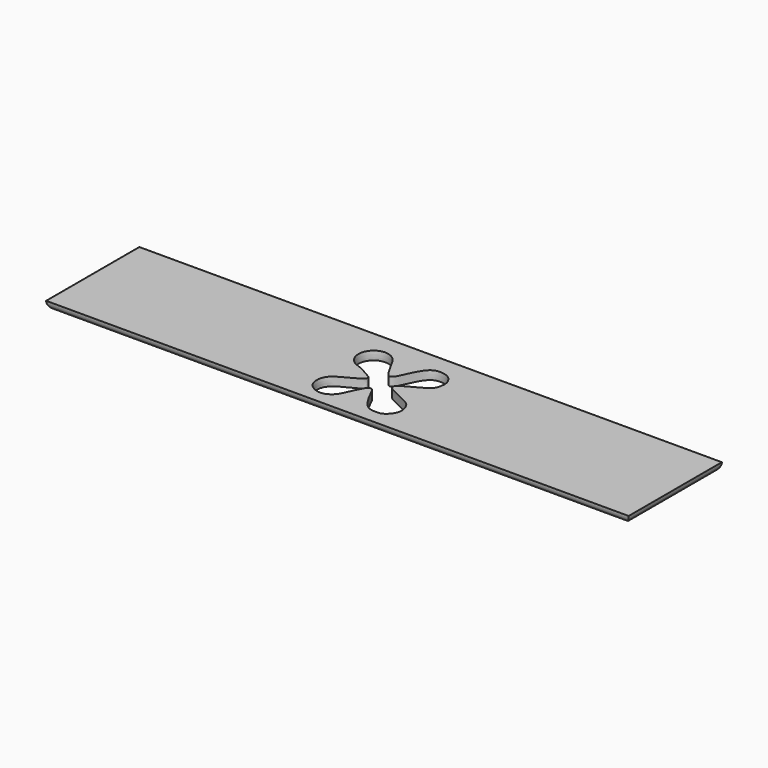
from build123d import *

# Parameters (mm, degrees)
F0_W        = 1282.7
F0_H        = 256.54
F1_DEPTH    = 19.1262
F2_R        = 19.0590813946
F3_T1_DEPTH = 1291.926483958
F3_T3_DEPTH = 265.766483958
F6_DEPTH    = 219.27551


# Not quite as in the source:
# - a fillet or chamfer that OpenCascade refuses, or shapes differently, is made with other operations: its cross-section is extruded or revolved along the edge and cut away or added


with BuildPart() as f1:
    # F0 (on Top) → F1 (new body)
    with BuildSketch(Plane.XY):
        with Locations((1.9049979746, -79.4771378769)):
            Rectangle(F0_W, F0_H)
    extrude(amount=F1_DEPTH)

    # F2
    f2_edges = [f1.edges().sort_by_distance(p)[0] for p in [
        (1.904998, -207.747138, 0),
        (-639.445002, -79.477138, 0),
        (1.904998, 48.792862, 0),
        (643.254998, -79.477138, 0),
    ]]
    fillet(f2_edges, radius=F2_R)

    # F3: fillet of radius 25.4 on 5 edges, made by hand

    # F3_s2 → F3_t1 (cut)
    with BuildSketch(Plane.YZ.offset(-644.0582440044)):
        with BuildLine():
            ThreePointArc((48.7928621231, 19.0590813946), (47.8708238484, 19.1094148025), (46.9475653315, 19.1262))
            Line((46.9475653315, 19.1262), (48.7928621231, 19.1262))
            Line((48.7928621231, 19.1262), (48.7928621231, 19.0590813946))
        make_face()
        with BuildLine():
            ThreePointArc((-205.9018410853, 19.1262), (-206.8250996022, 19.1094148025), (-207.7471378769, 19.0590813946))
            Line((-207.7471378769, 19.0590813946), (-207.7471378769, 19.1262))
            Line((-207.7471378769, 19.1262), (-205.9018410853, 19.1262))
        make_face()
    extrude(amount=F3_T1_DEPTH, mode=Mode.SUBTRACT)

    # F3_s4 → F3_t3 (cut)
    with BuildSketch(Plane.XZ.offset(-53.4061041021)):
        with BuildLine():
            ThreePointArc((-637.5997052338, 19.1262), (-638.5229637507, 19.1094148025), (-639.4450020254, 19.0590813946))
            Line((-639.4450020254, 19.0590813946), (-639.4450020254, 19.1262))
            Line((-639.4450020254, 19.1262), (-637.5997052338, 19.1262))
        make_face()
        with BuildLine():
            ThreePointArc((643.2549979746, 19.0590813946), (642.3329597, 19.1094148025), (641.409701183, 19.1262))
            Line((641.409701183, 19.1262), (643.2549979746, 19.1262))
            Line((643.2549979746, 19.1262), (643.2549979746, 19.0590813946))
        make_face()
    extrude(amount=F3_T3_DEPTH, mode=Mode.SUBTRACT)

    # F5 (on face) → F6 (cut)
    with BuildSketch(Plane.XY.offset(19.1262)):
        with BuildLine():
            add(Edge.make_bspline(
                [(-3.9519034326, -58.3399571478), (-6.0360933822, -57.4592299023), (-12.1793255374, -50.9473924507), (-26.2298304514, -24.3224308517), (-41.2097493794, 2.9789491334), (-72.4360201049, 10.037217761), (-96.3421712705, -9.9579243998), (-97.7950455083, -37.9438595198), (-81.6831294585, -58.938620379), (-61.293313593, -63.2792187165), (-36.9211355632, -78.9844871293), (-29.9788714537, -81.7077400378), (-25.2014666644, -91.8610913919), (-59.0203507366, -108.463960156), (-80.1276897444, -119.4826575733), (-93.5746327257, -137.4339169363), (-90.7677488387, -163.9002438236), (-75.433428627, -176.9677968773), (-53.4410245485, -183.5763107426), (-29.7456035179, -168.6651562344), (-22.0503636386, -143.9154043667), (-9.3604006708, -122.623140043), (-5.8408588762, -114.5198839058), (0.1862852859, -112.8583130861), (6.0845539399, -116.437681633), (11.1546658823, -128.0348941145), (35.0716542184, -175.5000656928), (59.8901853388, -176.6263497926), (75.1019291881, -176.9596767577), (92.8142614948, -159.8640561226), (94.7164382348, -139.7177878097), (85.5798052194, -118.6339024908), (64.9263701876, -110.1715280012), (41.5355938617, -97.6698881148), (26.6709534452, -91.1238108278), (23.6638573364, -79.4468287933), (58.8231521405, -61.5196046341), (86.0496608916, -47.4404865202), (89.3292768817, -29.5063854468), (90.8427014757, -17.0075569753), (83.8179274588, -3.1196709882), (72.876567362, 6.5813384408), (49.4892294606, 10.7817550348), (33.2966053013, 1.1094112138), (21.4575643669, -18.8380942056), (12.8511072657, -37.2941129706), (6.7906675389, -51.7553993461), (0.5542314898, -58.8191746249), (-2.616135601, -58.9044196736), (-3.9519034326, -58.3399571478)],
                knots=[0, 0, 0, 0, 0.0151229584, 0.0421015279, 0.0692616035, 0.0948049462, 0.1203362879, 0.1450368928, 0.1687479785, 0.1914131801, 0.2172722206, 0.2304272682, 0.2429599153, 0.2713252053, 0.2963517214, 0.3183061381, 0.3422399591, 0.3635317357, 0.3859579624, 0.4102418819, 0.4353682028, 0.4595571254, 0.473421007, 0.484424615, 0.4959678507, 0.5134155746, 0.5481570531, 0.5711454908, 0.5895783343, 0.6125261041, 0.634073892, 0.6563290025, 0.6791269627, 0.7046533686, 0.7237099907, 0.7369733968, 0.7666342284, 0.7940497901, 0.8134797873, 0.8305862037, 0.8491370062, 0.8676907375, 0.8905913388, 0.9111236605, 0.9343984251, 0.956730747, 0.9760954269, 0.9903076198, 1, 1, 1, 1], degree=3))
        make_face()
    extrude(amount=-F6_DEPTH, mode=Mode.SUBTRACT)


solid = f1.part
